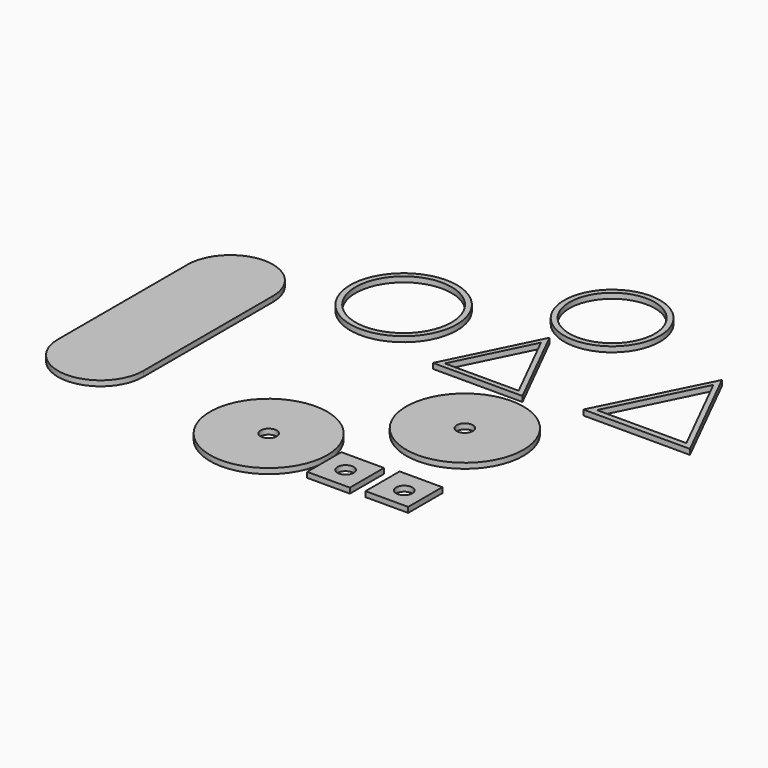
from build123d import *

# Parameters (mm, degrees)
F1_R      = 34.925
F1_R_2    = 4.826
F2_DEPTH  = 3.175
F3_R      = 34.925
F4_DEPTH  = 3.175
F5_R      = 4.826
F6_DEPTH  = 25.4
F7_W      = 25.4
F7_H      = 25.4
F7_R      = 4.826
F8_DEPTH  = 3.175
F0_R      = 31.75
F0_R_2    = 28.575
F9_DEPTH  = 3.175
F11_DEPTH = 3.175
F13_DEPTH = 3.175
F14_R     = 28.575
F14_R_2   = 25.4
F15_DEPTH = 3.175


# Not quite as in the source:
# - a feature names something its author has since deleted; it is built from what else it names


with BuildPart() as f2:
    # F1 (on Top) → F2 (new body)
    with BuildSketch(Plane.XY):
        with Locations((-41.45681113, -107.801027596)):
            Circle(F1_R)
        with Locations((-41.45681113, -107.801027596)):
            Circle(F1_R_2, mode=Mode.SUBTRACT)
    extrude(amount=F2_DEPTH)


with BuildPart() as f4:
    # F3 (on Top) → F4 (new body)
    with BuildSketch(Plane.XY):
        with Locations((26.4654487837, -46.6705858707)):
            Circle(F3_R)
    extrude(amount=F4_DEPTH)

    # F5 (on face) → F6 (cut)
    with BuildSketch(Plane.XY.offset(3.175)):
        with Locations((26.4654487837, -46.6705858707)):
            Circle(F5_R)
    extrude(amount=-F6_DEPTH, mode=Mode.SUBTRACT)


with BuildPart() as f8:
    # F7 (on Top) → F8 (new body)
    with BuildSketch(Plane.XY):
        with Locations((9.4302088464, -114.1496481273)):
            Rectangle(F7_W, F7_H)
        with Locations((9.4302088464, -114.1496481273)):
            Circle(F7_R, mode=Mode.SUBTRACT)
    extrude(amount=F8_DEPTH)


with BuildPart() as f8b:
    # F7 (on Top) → F8, piece 2 (new body)
    with BuildSketch(Plane.XY):
        with Locations((42.7242840971, -112.3598849141)):
            Rectangle(F7_W, F7_H)
        with Locations((43.6191657037, -113.2547665207)):
            Circle(F7_R, mode=Mode.SUBTRACT)
    extrude(amount=F8_DEPTH)


with BuildPart() as f9:
    # F0 (on Top) → F9 (new body)
    with BuildSketch(Plane.XY):
        with Locations((-73.4194368124, 32.6004140079)):
            Circle(F0_R)
        with Locations((-73.4194368124, 32.6004140079)):
            Circle(F0_R_2, mode=Mode.SUBTRACT)
    extrude(amount=F9_DEPTH)


with BuildPart() as f9b:
    # F0 (on Top) → F9, piece 2 (new body)
    with BuildSketch(Plane.XY):
        Polygon((89.5012710243, 65.8874005459), (57.7512710243, 2.3874005459), (121.2512710243, 2.3874005459), align=None)
        Polygon((116.3342488013, 5.871444992), (63.0601253544, 5.871444992), (89.5012710243, 59.5374005459), align=None, mode=Mode.SUBTRACT)
    extrude(amount=F9_DEPTH)


with BuildPart() as f11:
    # F10 (on Top) → F11 (new body)
    with BuildSketch(Plane.XY):
        with BuildLine():
            Line((-126.3140311956, -95.0520038605), (-126.3140311956, 1.4679961395))
            ThreePointArc((-126.3140311956, 1.4679961395), (-151.7140311956, 26.8679961395), (-177.1140311956, 1.4679961395))
            Line((-177.1140311956, 1.4679961395), (-177.1140311956, -95.0520038605))
            ThreePointArc((-177.1140311956, -95.0520038605), (-151.7140311956, -120.4520038605), (-126.3140311956, -95.0520038605))
        make_face()
    extrude(amount=F11_DEPTH)


with BuildPart() as f13:
    # F12 (on Top) → F13 (new body)
    with BuildSketch(Plane.XY):
        Polygon((0.3149577829, 49.0201465513), (-26.1261878871, -4.6458090026), (27.1479355598, -4.6458090026), align=None)
        Polygon((-21.5025167309, -1.6114300556), (0.3149577829, 42.6701465513), (22.4557460863, -1.6114300556), align=None, mode=Mode.SUBTRACT)
    extrude(amount=F13_DEPTH)


with BuildPart() as f15:
    # F14 (on Top) → F15 (new body)
    with BuildSketch(Plane.XY):
        with Locations((10.6468005106, 82.7375650406)):
            Circle(F14_R)
        with Locations((10.6468005106, 82.7375650406)):
            Circle(F14_R_2, mode=Mode.SUBTRACT)
    extrude(amount=F15_DEPTH)


solid = Compound([f2.part, f4.part, f8.part, f8b.part, f9.part, f9b.part, f11.part, f13.part, f15.part])
